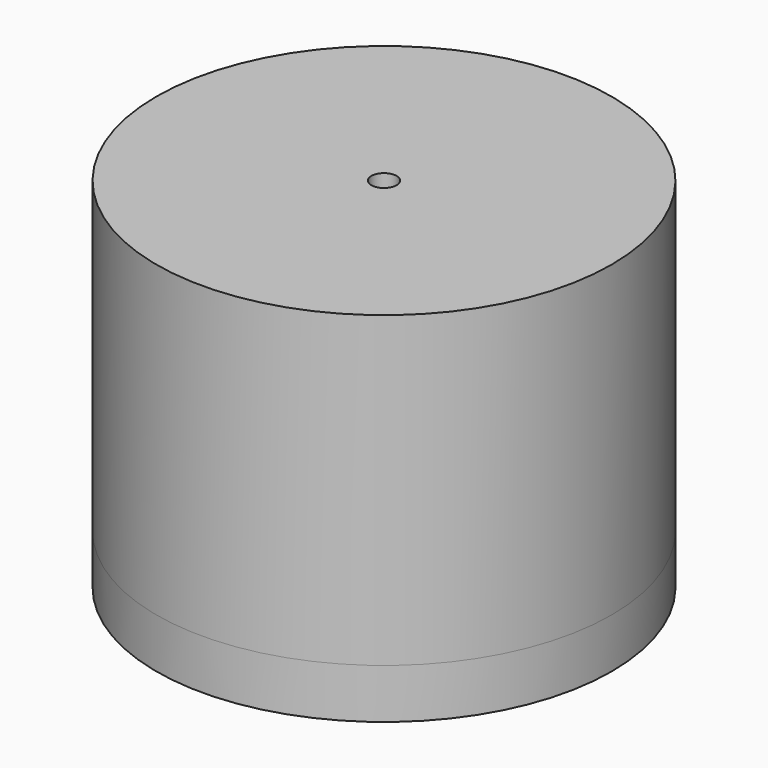
from build123d import *


# Not quite as in the source:
# - ends of sketch curves that miss each other by under 0.0002 mm in the source are joined


with BuildPart() as f1:
    # F0 (on Front) → F1 (revolve)
    with BuildSketch(Plane.XZ):
        with BuildLine():
            Line((-5.5049625925, 43.2034109984), (-5.5049625925, 83.3543194161))
            Line((-5.5049625925, 83.3543194161), (-99.4309840389, 83.3543194161))
            Line((-99.4309840389, 83.3543194161), (-99.4309840389, -51.3714465576))
            Line((-99.4309840389, -51.3714465576), (-87.4468881672, -51.3714465576))
            Line((-87.4468881672, -51.3714465576), (-87.4468881672, -39.1072945867))
            Line((-87.4468881672, -39.1072945867), (-79.5739456842, -39.1072945867))
            Line((-79.5739456842, -39.1072945867), (-79.5739456842, -51.3714465576))
            Line((-79.5739456842, -51.3714465576), (-64.008, -51.3714465576))
            add(Edge.make_bspline(
                [(-64.008, -51.3714465576), (-64.1027038454, -49.839950803), (-62.7670473342, -44.0198094824), (-59.795903973, -40.557544581), (-54.6012246924, -36.8234386179), (-49.7372082623, -32.6662543777), (-46.8715955049, -26.175741387), (-43.5946465593, -19.1096878414), (-41.7681298564, -8.6181796833), (-40.0560318039, -0.0270351042), (-37.2140229768, 20.4769103307), (-34.5096956961, 33.4115075529), (-28.8439262592, 41.7285244533), (-17.6651301621, 42.8076889627), (-5.5049625925, 43.2034109984)],
                knots=[0, 0, 0, 0, 0.0708281388, 0.1296061177, 0.1961624378, 0.26371795, 0.3337316046, 0.4090991647, 0.494396835, 0.5753960354, 0.6970604735, 0.79528122, 0.8698391379, 1, 1, 1, 1], degree=3))
        make_face()
    revolve(axis=Axis((0, 0, -9.7730937459), (0, 0, -1)))


with BuildPart() as f3:
    # F2 (on Front) → F3 (revolve)
    with BuildSketch(Plane.XZ):
        with BuildLine():
            add(Edge.make_bspline(
                [(-64.008, -51.3714570016), (-62.1417719206, -51.1193087771), (-58.2184243409, -50.6835159057), (-54.80499818, -48.0288890525), (-50.869415203, -44.8556398767), (-44.9076833426, -38.6843511379), (-41.1418422638, -28.5836251876), (-36.8837585479, -11.3600621188), (-35.5512845454, 3.654102122), (-32.5751230407, 21.3452100724), (-31.6428957309, 28.546524663), (-28.6921245131, 33.535284546), (-26.2962108333, 35.7112909355), (-19.4360185112, 37.9818852252), (-10.8556993698, 38.9875847862), (-3.7151385315, 39.0980221276), (0, 39.1552485526)],
                knots=[0, 0, 0, 0, 0.0585835377, 0.1084324952, 0.1630098689, 0.2330534173, 0.3136392856, 0.4158345544, 0.5140429199, 0.6166278982, 0.6829616528, 0.7389680389, 0.7822413443, 0.8461057652, 0.9191022622, 1, 1, 1, 1], degree=3))
            Line((-64.008, -51.3714570016), (-16.9247925652, -51.1193087771))
            Line((-16.9247925652, -51.1193087771), (-16.9452934719, -47.2912094683))
            Line((-16.9452934719, -47.2912094683), (-8.3812896029, -47.2453460174))
            Line((-8.3812896029, -47.2453460174), (-8.3605430802, -51.1193087771))
            Line((-8.3605430802, -51.1193087771), (0, -51.074534935))
            Line((0, -51.074534935), (0, 39.1552485526))
        make_face()
    revolve(axis=Axis((0, 0, -5.9596431912), (0, 0, 1)))


with BuildPart() as f5:
    # F4 (on Front) → F5 (revolve)
    with BuildSketch(Plane.XZ):
        Polygon((-87.4468881672, -51.3714465576), (-99.4309840389, -51.3714465576), (-99.4309840389, -73.1087177992), (0, -73.1087177992), (0, -51.074534935), (-8.3605430802, -51.1193087771), (-8.3812896029, -47.2453460174), (-16.9452934719, -47.2912094683), (-16.9247925652, -51.1193087771), (-64.008, -51.3714570016), (-79.5739456842, -51.3714465576), (-79.5739456842, -39.1072945867), (-87.4468881672, -39.1072945867), align=None)
    revolve(axis=Axis((0, 0, -120.2870681882), (0, 0, -1)))


solid = Compound([f1.part, f3.part, f5.part])
